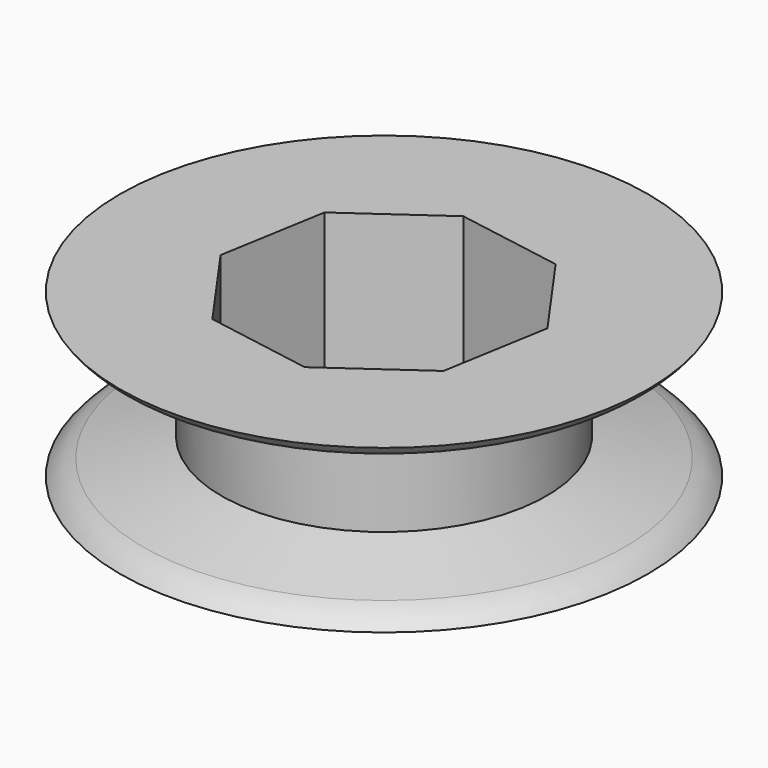
from build123d import *

# Parameters (mm, degrees)
F4_DEPTH = 8.001


# Not quite as in the source:
# - a fillet or chamfer that OpenCascade refuses, or shapes differently, is made with other operations: its cross-section is extruded or revolved along the edge and cut away or added


with BuildPart() as f1:
    # F0 (on Front) → F1 (revolve)
    with BuildSketch(Plane.XZ):
        Polygon((-13, 0), (0, 0), (0, 8), (-13, 8), (-13, 7.5), (-8, 6.25), (-8, 1.75), (-13, 0.5), align=None)
    revolve(axis=Axis((0, 0, 4), (0, 0, 1)))

    # F2: fillet of radius 2 on 2 edges, made by hand

    # F2_s1 → F2_t2 (revolve, cut)
    with BuildSketch(Plane.XZ):
        with BuildLine():
            ThreePointArc((-13, 8), (-12.4961942947, 7.5030870148), (-11.8508805842, 7.212720146))
            Line((-11.8508805842, 7.212720146), (-13, 7.5))
            Line((-13, 7.5), (-13, 8))
        make_face()
    revolve(axis=Axis((0, 0, 7.5), (0, 0, 1)), mode=Mode.SUBTRACT)

    # F2_s3 → F2_t4 (revolve, cut)
    with BuildSketch(Plane.XZ):
        with BuildLine():
            ThreePointArc((-11.8508805842, 0.787279854), (-12.4961942947, 0.4969129852), (-13, 0))
            Line((-13, 0), (-13, 0.5))
            Line((-13, 0.5), (-11.8508805842, 0.787279854))
        make_face()
    revolve(axis=Axis((0, 0, 0.5), (0, 0, 1)), mode=Mode.SUBTRACT)

    # F3 (on Top) → F4 (cut, through all)
    with BuildSketch(Plane.XY):
        Polygon((6.808574619, 1.5439145703), (3.722676821, 5.9061017456), (-1.5439145703, 6.808574619), (-5.9061017456, 3.722676821), (-6.808574619, -1.5439145703), (-3.722676821, -5.9061017456), (1.5439145703, -6.808574619), (5.9061017456, -3.722676821), align=None)
    extrude(amount=F4_DEPTH, mode=Mode.SUBTRACT)


solid = f1.part
